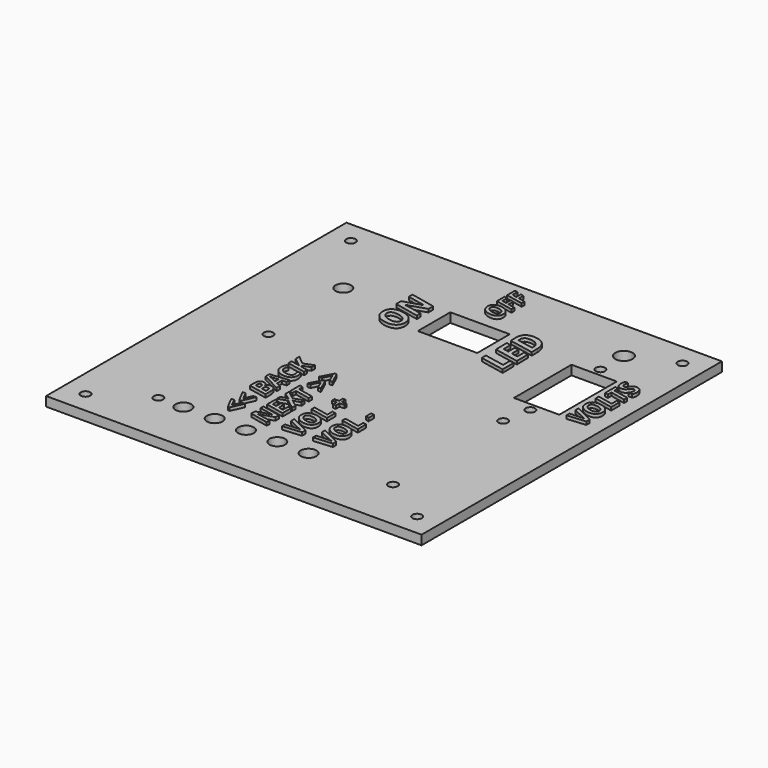
from build123d import *

# Parameters (mm, degrees)
F0_W          = 120
F0_H          = 120
F0_R          = 1.5
F1_DEPTH      = 3
F5_TEXT_SIZE  = 8.3333333333
F6_DEPTH      = 1
F7_TEXT_SIZE  = 8.3333333333
F8_DEPTH      = 1
F9_TEXT_SIZE  = 8.3333333333
F10_DEPTH     = 1
F11_TEXT_SIZE = 8.3333333333
F12_DEPTH     = 1
F13_DEPTH     = 4
F2_R          = 1.5
F2_R_2        = 2.5
F2_W          = 19
F2_H          = 13
F14_DEPTH     = 3
F15_TEXT_SIZE = 11.1111111111
F16_DEPTH     = 1
F17_TEXT_SIZE = 11.1111111111
F18_DEPTH     = 1
F19_DEPTH     = 5
F20_TEXT_SIZE = 7.7670698043
F21_DEPTH     = 1
F22_W         = 14.5
F22_H         = 23
F22_R         = 1.5
F22_R_2       = 2.75
F23_DEPTH     = 5
F24_TEXT_SIZE = 8.3333333333
F25_DEPTH     = 1
F26_R         = 2.5
F27_DEPTH     = 5


# Not quite as in the source:
# - the program builds the solid bodies; features that only make, move or delete a surface that nothing else refers to are left out
# - Text() gives the source's letters only with a copy of the font that has no kerning and outlines rounded to 1/6400 em; it was checked with that copy


with BuildPart() as f1:
    # F0 (on Top) → F1 (new body)
    with BuildSketch(Plane.XY):
        Rectangle(F0_W, F0_H)
        with Locations((-53, -53)):
            Circle(F0_R, mode=Mode.SUBTRACT)
        with Locations((53, -53)):
            Circle(F0_R, mode=Mode.SUBTRACT)
        with Locations((-53, 53)):
            Circle(F0_R, mode=Mode.SUBTRACT)
        with Locations((53, 53)):
            Circle(F0_R, mode=Mode.SUBTRACT)
    extrude(amount=F1_DEPTH)

    # F5 (on face) → F6 (join)
    with BuildSketch(Plane.XY.offset(3)):
        with Locations(Location((-16.5656337361, -38.0849085928), (0, 0, 90.3587429475))):
            Text('<< BACK', F5_TEXT_SIZE, font='Open Sans', font_style=FontStyle.BOLDITALIC, text_align=(TextAlign.LEFT, TextAlign.BOTTOM))
    extrude(amount=F6_DEPTH)

    # F7 (on face) → F8 (join)
    with BuildSketch(Plane.XY.offset(3)):
        with Locations(Location((-6.9628858164, -38.3672978889), (0, 0, 89.9267305325))):
            Text('NEXT >>', F7_TEXT_SIZE, font='Open Sans', font_style=FontStyle.BOLDITALIC, text_align=(TextAlign.LEFT, TextAlign.BOTTOM))
    extrude(amount=F8_DEPTH)

    # F9 (on face) → F10 (join)
    with BuildSketch(Plane.XY.offset(3)):
        with Locations(Location((3.324544372, -38.167979721), (0, 0, 90.0068338533))):
            Text('VOL +', F9_TEXT_SIZE, font='Open Sans', font_style=FontStyle.BOLDITALIC, text_align=(TextAlign.LEFT, TextAlign.BOTTOM))
    extrude(amount=F10_DEPTH)

    # F11 (on face) → F12 (join)
    with BuildSketch(Plane.XY.offset(3)):
        with Locations(Location((13.1265195237, -38.1137250591), (0, 0, 89.9300926975))):
            Text('VOL -', F11_TEXT_SIZE, font='Open Sans', font_style=FontStyle.BOLDITALIC, text_align=(TextAlign.LEFT, TextAlign.BOTTOM))
    extrude(amount=F12_DEPTH)

    # F0 (on Top) → F13 (cut)
    with BuildSketch(Plane.XY):
        Rectangle(F0_W, F0_H)
        with Locations((-53, -53)):
            Circle(F0_R, mode=Mode.SUBTRACT)
        with Locations((53, -53)):
            Circle(F0_R, mode=Mode.SUBTRACT)
        with Locations((-53, 53)):
            Circle(F0_R, mode=Mode.SUBTRACT)
        with Locations((53, 53)):
            Circle(F0_R, mode=Mode.SUBTRACT)
    extrude(amount=-F13_DEPTH, mode=Mode.SUBTRACT)

    # F2 (on face) → F14 (cut)
    with BuildSketch(Plane.XY.offset(3)):
        with Locations((-37.5, 0.7379425162)):
            Circle(F2_R)
        with Locations((37.5, 0.7379425162)):
            Circle(F2_R)
        with Locations((37.5, -43.2620574838)):
            Circle(F2_R)
        with Locations((-37.5, -43.2620574838)):
            Circle(F2_R)
        with Locations((-29.5, -43.2620574838)):
            Circle(F2_R_2)
        with Locations((-19.5, -43.2620574838)):
            Circle(F2_R_2)
        with Locations((-9.5, -43.2620574838)):
            Circle(F2_R_2)
        with Locations((0.5, -43.2620574838)):
            Circle(F2_R_2)
        with Locations((10.5, -43.2620574838)):
            Circle(F2_R_2)
        with Locations((0, 31.8677723408)):
            Rectangle(F2_W, F2_H)
    extrude(amount=-F14_DEPTH, mode=Mode.SUBTRACT)

    # F15 (on face) → F16 (join)
    with BuildSketch(Plane.XY.offset(3)):
        with Locations(Location((-13.7386224715, 21.8515595875), (0, 0, 89.839304368))):
            Text('ON', F15_TEXT_SIZE, font='Open Sans', font_style=FontStyle.BOLDITALIC, text_align=(TextAlign.LEFT, TextAlign.BOTTOM))
    extrude(amount=F16_DEPTH)

    # F17 (on face) → F18 (join)
    with BuildSketch(Plane.XY.offset(3)):
        with Locations(Location((21.1888219495, 20.6583521647), (0, 0, 90.7631165423))):
            Text('LED', F17_TEXT_SIZE, font='Open Sans', font_style=FontStyle.BOLDITALIC, text_align=(TextAlign.LEFT, TextAlign.BOTTOM))
    extrude(amount=F18_DEPTH)

    # F2 (on face) → F19 (cut)
    with BuildSketch(Plane.XY.offset(3)):
        with Locations((-37.5, 0.7379425162)):
            Circle(F2_R)
        with Locations((37.5, 0.7379425162)):
            Circle(F2_R)
        with Locations((37.5, -43.2620574838)):
            Circle(F2_R)
        with Locations((-37.5, -43.2620574838)):
            Circle(F2_R)
        with Locations((-29.5, -43.2620574838)):
            Circle(F2_R_2)
        with Locations((-19.5, -43.2620574838)):
            Circle(F2_R_2)
        with Locations((-9.5, -43.2620574838)):
            Circle(F2_R_2)
        with Locations((0.5, -43.2620574838)):
            Circle(F2_R_2)
        with Locations((10.5, -43.2620574838)):
            Circle(F2_R_2)
        with Locations((0, 31.8677723408)):
            Rectangle(F2_W, F2_H)
    extrude(amount=-F19_DEPTH, mode=Mode.SUBTRACT)

    # F20 (on face) → F21 (join)
    with BuildSketch(Plane.XY.offset(3)):
        with Locations(Location((2.5914413854, 41.7996942997), (0, 0, 90.1305299814))):
            Text('OFF', F20_TEXT_SIZE, font='Open Sans', font_style=FontStyle.BOLDITALIC, text_align=(TextAlign.LEFT, TextAlign.BOTTOM))
    extrude(amount=F21_DEPTH)

    # F22 (on face) → F23 (cut)
    with BuildSketch(Plane.XY.offset(3)):
        with Locations((39.0726478994, 23.613568373)):
            Rectangle(F22_W, F22_H)
        with Locations((39.0726478994, 9.613568373)):
            Circle(F22_R)
        with Locations((39.0726478994, 37.613568373)):
            Circle(F22_R)
        with Locations((39.0726478994, 47)):
            Circle(F22_R_2)
    extrude(amount=-F23_DEPTH, mode=Mode.SUBTRACT)

    # F24 (on face) → F25 (join)
    with BuildSketch(Plane.XY.offset(3)):
        with Locations(Location((55.0718313767, 10.7258790968), (0, 0, 90.0843837548))):
            Text('VOLTS', F24_TEXT_SIZE, font='Open Sans', font_style=FontStyle.BOLDITALIC, text_align=(TextAlign.LEFT, TextAlign.BOTTOM))
    extrude(amount=F25_DEPTH)

    # F26 (on face) → F27 (cut)
    with BuildSketch(Plane.XY.offset(3)):
        with Locations((-38.4977087379, 31.8677723408)):
            Circle(F26_R)
    extrude(amount=-F27_DEPTH, mode=Mode.SUBTRACT)


solid = f1.part
